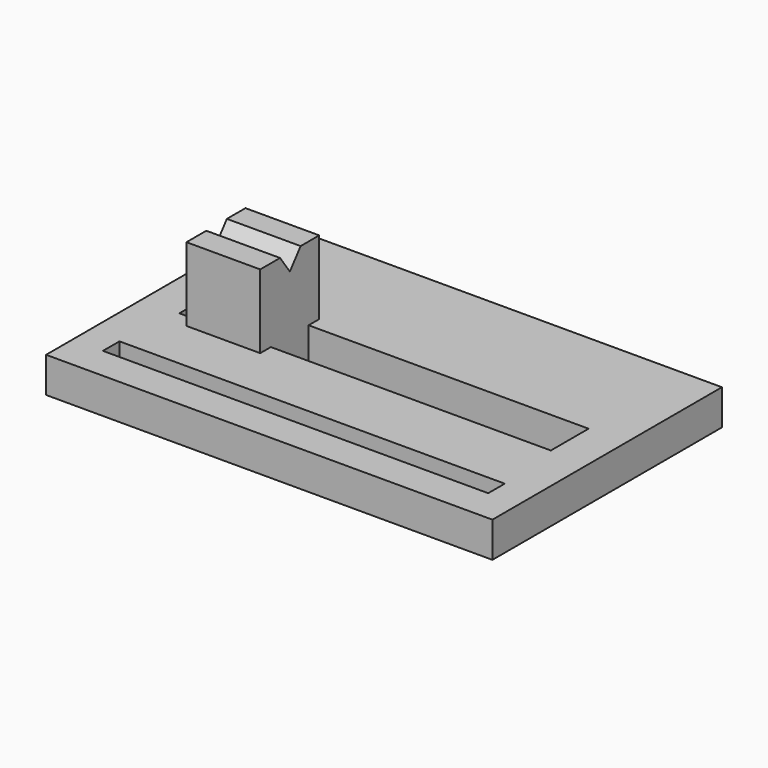
from build123d import *

# Parameters (mm, degrees)
F0_W     = 151.3114133903
F0_H     = 97.2457080337
F0_W_2   = 130.6122839451
F0_H_2   = 7.0094466209
F0_W_3   = 25
F0_H_3   = 4
F0_H_4   = 0.5
F1_DEPTH = 12
F0_H_5   = 16
F2_DEPTH = 25
F3_DEPTH = 12
F5_DEPTH = 25


with BuildPart() as f1:
    # F0 (on Top) → F1 (new body)
    with BuildSketch(Plane.XY):
        Rectangle(F0_W, F0_H)
        with Locations((0, -33.9665152133)):
            Rectangle(F0_W_2, F0_H_2, mode=Mode.SUBTRACT)
        Polygon((-66.2499921114, 12), (-56.9642793678, 12), (-56.9642793678, 12.5), (-31.9642793678, 12.5), (-31.9642793678, 12), (66.2499921114, 12), (66.2499921114, -12), (-31.9642793678, -12), (-31.9642793678, -12.5), (-56.9642793678, -12.5), (-56.9642793678, -12), (-66.2499921114, -12), align=None, mode=Mode.SUBTRACT)
        with Locations((-44.4642793678, 10)):
            Rectangle(F0_W_3, F0_H_3)
        Polygon((-62.9557022443, -8), (-62.9557022443, 8), (-56.9642793678, 8), (-56.9642793678, 12), (-66.2499921114, 12), (-66.2499921114, -12), (-56.9642793678, -12), (-56.9642793678, -8), align=None)
        with Locations((-44.4642793678, 12.25)):
            Rectangle(F0_W_3, F0_H_4)
        with Locations((-44.4642793678, -10)):
            Rectangle(F0_W_3, F0_H_3)
        with Locations((-44.4642793678, -12.25)):
            Rectangle(F0_W_3, F0_H_4)
        Polygon((-31.9642793678, 12), (-31.9642793678, 8), (62.9557022443, 8), (62.9557022443, -8), (-31.9642793678, -8), (-31.9642793678, -12), (66.2499921114, -12), (66.2499921114, 12), align=None)
    extrude(amount=-F1_DEPTH)


with BuildPart() as f2:
    # F0 (on Top) → F2 (new body)
    with BuildSketch(Plane.XY):
        with Locations((-44.4642793678, -12.25)):
            Rectangle(F0_W_3, F0_H_4)
        with Locations((-44.4642793678, -10)):
            Rectangle(F0_W_3, F0_H_3)
        with Locations((-44.4642793678, 0)):
            Rectangle(F0_W_3, F0_H_5)
        with Locations((-44.4642793678, 10)):
            Rectangle(F0_W_3, F0_H_3)
        with Locations((-44.4642793678, 12.25)):
            Rectangle(F0_W_3, F0_H_4)
    extrude(amount=F2_DEPTH)

    # F0 (on Top) → F3 (join, through all)
    with BuildSketch(Plane.XY):
        with Locations((-44.4642793678, 0)):
            Rectangle(F0_W_3, F0_H_5)
    extrude(amount=-F3_DEPTH)

    # F4 (on face) → F5 (cut)
    with BuildSketch(Plane(origin=(-56.9642793678, 0, 0), x_dir=(0, -1, 0), z_dir=(-1, 0, 0))):
        Polygon((4.0890707848, 25), (-4.6258270741, 25), (-0.0637064282, 19.2482927877), align=None)
    extrude(amount=-F5_DEPTH, mode=Mode.SUBTRACT)


solid = Compound([f1.part, f2.part])
